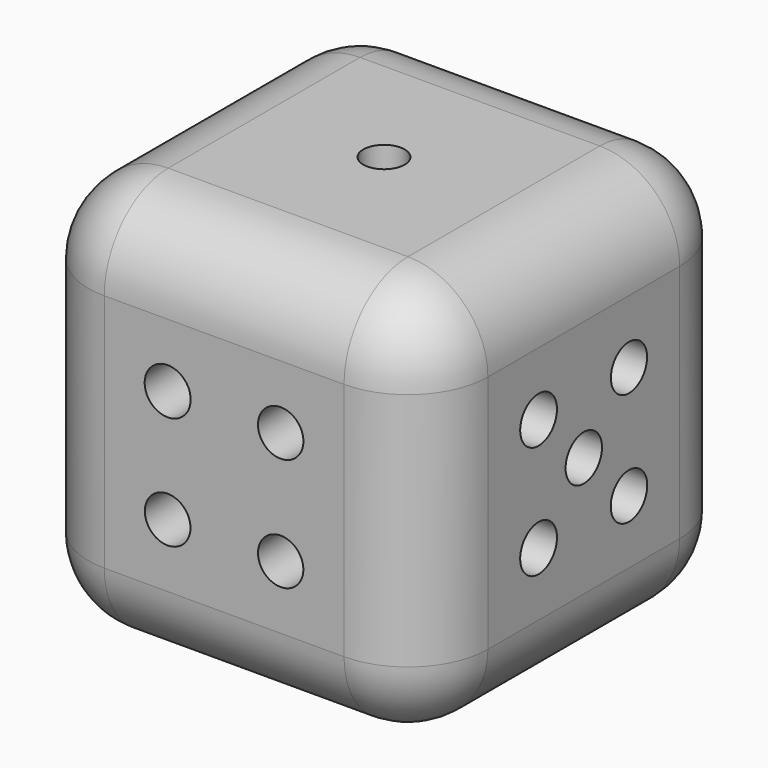
from build123d import *

# Parameters (mm, degrees)
F0_W      = 63.5
F0_H      = 63.5
F1_DEPTH  = 63.5
F2_R      = 12.7
F3_R      = 3.2855032165
F4_DEPTH  = 10.16
F5_R      = 5.08
F6_DEPTH  = 2.54
F7_R      = 4.1642644098
F7_R_2    = 3.880802303
F8_DEPTH  = 10.16
F9_R      = 3.6538042468
F9_R_2    = 3.616555367
F9_R_3    = 3.5948118785
F9_R_4    = 3.6557525946
F9_R_5    = 3.6263948518
F10_DEPTH = 10.16
F11_R     = 3.6080090175
F11_R_2   = 3.6165563664
F11_R_3   = 3.6112952818
F12_DEPTH = 10.16
F13_R     = 3.6544564118
F13_R_2   = 3.6098297146
F13_R_3   = 3.6228239361
F13_R_4   = 3.6044825881
F14_DEPTH = 10.16


# Not quite as in the source:
# - a feature names something its author has since deleted; it is built from what else it names


with BuildPart() as f1:
    # F0 (on Top) → F1 (new body)
    with BuildSketch(Plane.XY):
        with Locations((-105.7584263082, 32.8302064445)):
            Rectangle(F0_W, F0_H)
    extrude(amount=F1_DEPTH)

    # F2
    f2_edges = [f1.edges().sort_by_distance(p)[0] for p in [
        (-74.008426, 32.830206, 0),
        (-137.508426, 32.830206, 0),
        (-105.758426, 1.080206, 0),
        (-137.508426, 1.080206, 31.75),
        (-74.008426, 1.080206, 31.75),
        (-137.508426, 32.830206, 63.5),
        (-105.758426, 64.580206, 0),
        (-137.508426, 64.580206, 31.75),
        (-105.758426, 64.580206, 63.5),
        (-74.008426, 64.580206, 31.75),
        (-74.008426, 32.830206, 63.5),
        (-105.758426, 1.080206, 63.5),
    ]]
    fillet(f2_edges, radius=F2_R)

    # F3 (on face) → F4 (cut)
    with BuildSketch(Plane.XY.offset(63.5)):
        with Locations((-105.7584263082, 32.8302064445)):
            Circle(F3_R)
    extrude(amount=-F4_DEPTH, mode=Mode.SUBTRACT)

    # F5 (on face) → F6 (cut)
    with BuildSketch(Plane(origin=(0, 0, 0), x_dir=(1, 0, 0), z_dir=(0, 0, -1))):
        with Locations((-111.8508055806, -21.4002064445)):
            Circle(F5_R)
        with Locations((-98.9837050438, -21.4002064445)):
            Circle(F5_R)
        with Locations((-111.8508055806, -32.8302064445)):
            Circle(F5_R)
        with Locations((-98.9837050438, -32.8302064445)):
            Circle(F5_R)
        with Locations((-111.8508055806, -44.2602064445)):
            Circle(F5_R)
        with Locations((-98.9837050438, -44.2602064445)):
            Circle(F5_R)
    extrude(amount=-F6_DEPTH, mode=Mode.SUBTRACT)

    # F7 (on face) → F8 (cut)
    with BuildSketch(Plane(origin=(-137.5084263082, 0, 0), x_dir=(0, -1, 0), z_dir=(-1, 0, 0))):
        with Locations((-40.1898002429, 39.1095937984)):
            Circle(F7_R)
        with Locations((-27.4898002429, 26.4095937984)):
            Circle(F7_R_2)
    extrude(amount=-F8_DEPTH, mode=Mode.SUBTRACT)

    # F9 (on face) → F10 (cut)
    with BuildSketch(Plane.YZ.offset(-74.0084263082)):
        with Locations((23.8499503234, 40.7302561211)):
            Circle(F9_R)
        with Locations((32.8302064445, 31.75)):
            Circle(F9_R_2)
        with Locations((41.8104625656, 40.7302561211)):
            Circle(F9_R_3)
        with Locations((23.8499503234, 22.7697438789)):
            Circle(F9_R_4)
        with Locations((41.8104625656, 22.7697438789)):
            Circle(F9_R_5)
    extrude(amount=-F10_DEPTH, mode=Mode.SUBTRACT)

    # F11 (on face) → F12 (cut)
    with BuildSketch(Plane(origin=(0, 64.5802064445, 0), x_dir=(-1, 0, 0), z_dir=(0, 1, 0))):
        with Locations((96.7781701871, 40.7302561211)):
            Circle(F11_R)
        with Locations((114.7386824292, 22.7697438789)):
            Circle(F11_R_2)
        with Locations((105.7584263082, 31.75)):
            Circle(F11_R_3)
    extrude(amount=-F12_DEPTH, mode=Mode.SUBTRACT)

    # F13 (on face) → F14 (cut)
    with BuildSketch(Plane.XZ.offset(-1.0802064445)):
        with Locations((-114.7386824292, 40.7302561211)):
            Circle(F13_R)
        with Locations((-96.7781701871, 40.7302561211)):
            Circle(F13_R_2)
        with Locations((-114.7386824292, 22.7697438789)):
            Circle(F13_R_3)
        with Locations((-96.7781701871, 22.7697438789)):
            Circle(F13_R_4)
    extrude(amount=-F14_DEPTH, mode=Mode.SUBTRACT)


solid = f1.part
